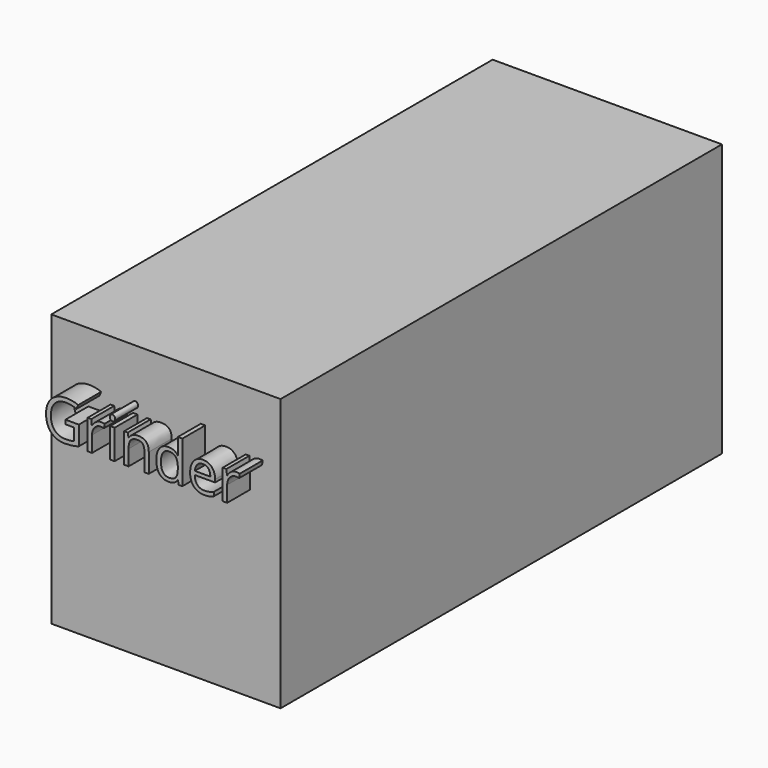
from build123d import *

# Parameters (mm, degrees)
F0_W         = 203.2
F0_H         = 241.3
F1_DEPTH     = 488.95
F2_TEXT_SIZE = 48.9028320942
F3_DEPTH     = 25.4


# Not quite as in the source:
# - Text() gives the source's letters only with a copy of the font that has no kerning and outlines rounded to 1/6400 em; it was checked with that copy


with BuildPart() as f1:
    # F0 (on Front) → F1 (new body)
    with BuildSketch(Plane.XZ):
        Rectangle(F0_W, F0_H)
    extrude(amount=F1_DEPTH)

    # F2 (on face) → F3 (join)
    with BuildSketch(Plane.XZ.offset(488.95)):
        with Locations((-88.9, 41.2459115074)):
            Text('Grinder', F2_TEXT_SIZE, font='Open Sans', text_align=(TextAlign.LEFT, TextAlign.BOTTOM))
    extrude(amount=F3_DEPTH)


solid = f1.part
